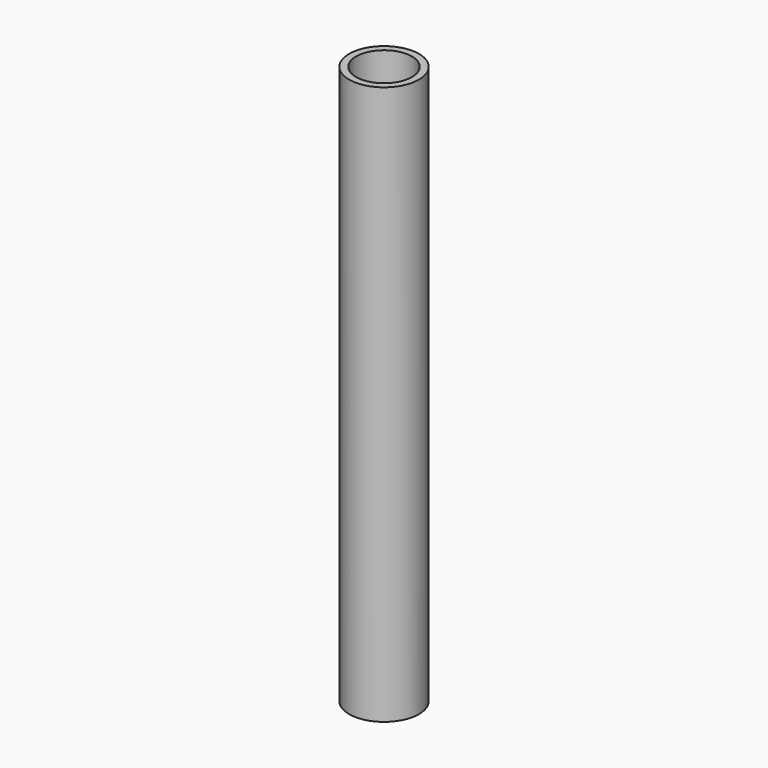
from build123d import *

# Parameters (mm, degrees)
F0_R     = 7.9375
F0_R_2   = 6.35
F1_DEPTH = 127


# Not quite as in the source:
# - a feature names something its author has since deleted; it is built from what else it names


with BuildPart() as f1:
    # F0 (on Top) → F1 (new body)
    with BuildSketch(Plane.XY):
        Circle(F0_R)
        Circle(F0_R_2, mode=Mode.SUBTRACT)
    extrude(amount=F1_DEPTH)


solid = f1.part
